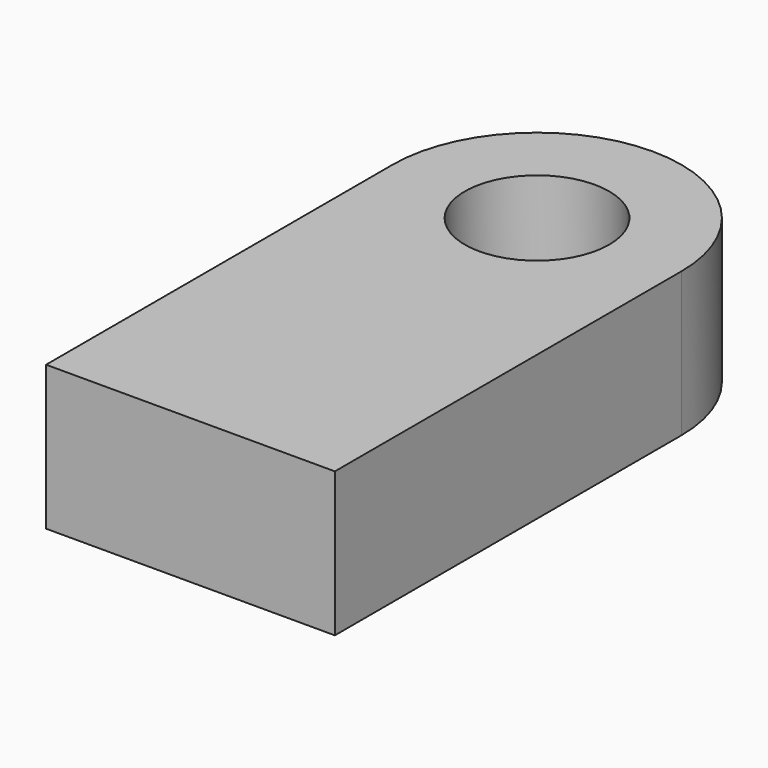
from build123d import *

# Parameters (mm, degrees)
F1_DEPTH = 25.4
F2_R     = 12.7
F3_DEPTH = 25.4


with BuildPart() as f1:
    # F0 (on Top) → F1 (new body)
    with BuildSketch(Plane.XY):
        with BuildLine():
            Line((-25.4, 76.2), (-25.4, 0))
            Line((-25.4, 0), (25.4, 0))
            Line((25.4, 0), (25.4, 76.2))
            ThreePointArc((25.4, 76.2), (0, 50.8), (-25.4, 76.2))
        make_face()
        with BuildLine():
            ThreePointArc((25.4, 76.2), (0, 101.6), (-25.4, 76.2))
            Line((-25.4, 76.2), (25.4, 76.2))
        make_face()
        with BuildLine():
            Line((25.4, 76.2), (-25.4, 76.2))
            ThreePointArc((-25.4, 76.2), (0, 50.8), (25.4, 76.2))
        make_face()
    extrude(amount=F1_DEPTH)

    # F2 (on face) → F3 (cut)
    with BuildSketch(Plane.XY.offset(25.4)):
        with Locations((0, 76.2)):
            Circle(F2_R)
    extrude(amount=-F3_DEPTH, mode=Mode.SUBTRACT)


solid = f1.part
